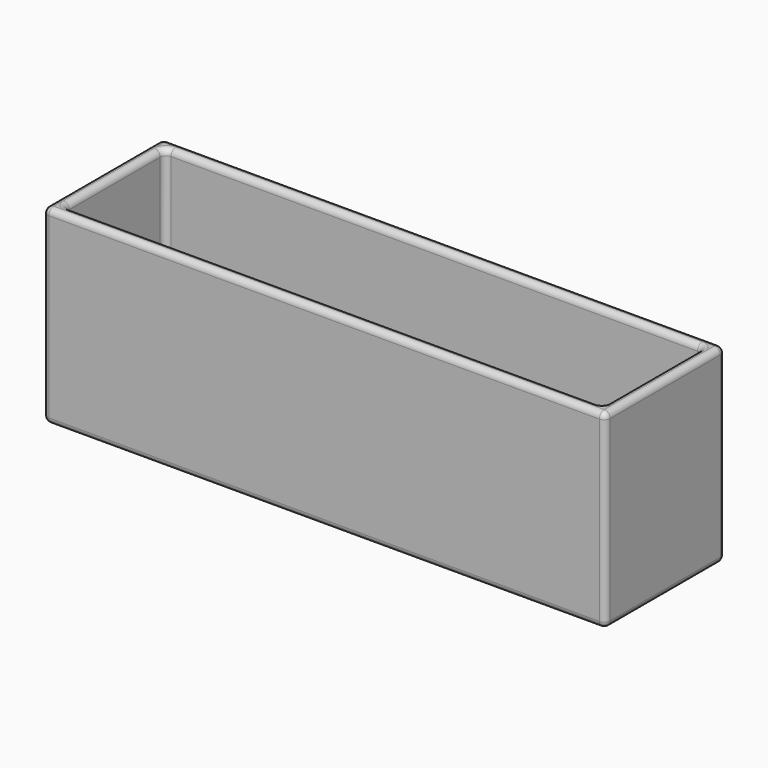
from build123d import *

# Parameters (mm, degrees)
F0_W     = 188
F0_H     = 63.5
F1_DEPTH = 50
F2_W     = 180
F2_H     = 42
F3_DEPTH = 59.5
F4_R     = 20
F5_DEPTH = 20
F6_R     = 7
F7_R     = 1.99999


# Not quite as in the source:
# - a fillet or chamfer is up to 0.001 mm smaller than in the source, because OpenCascade refuses the exact size


with BuildPart() as f1:
    # F0 (on Front) → F1 (new body)
    with BuildSketch(Plane.XZ):
        with Locations((31.2486086041, -31.75)):
            Rectangle(F0_W, F0_H)
    extrude(amount=F1_DEPTH)

    # F2 (on Top) → F3 (cut)
    with BuildSketch(Plane.XY):
        with Locations((31.2486086041, -25)):
            Rectangle(F2_W, F2_H)
    extrude(amount=-F3_DEPTH, mode=Mode.SUBTRACT)

    # F4 (on Front) → F5 (join)
    with BuildSketch(Plane.XZ):
        with Locations((31.2486086041, -31.75)):
            Circle(F4_R)
    extrude(amount=-F5_DEPTH)

    # F6
    f6_edges = [f1.edges().sort_by_distance(p)[0] for p in [
        (11.248609, 20, -31.75),
    ]]
    fillet(f6_edges, radius=F6_R)

    # F7 (radius 2 in the source; OpenCascade refuses exactly that, so slightly less here)
    f7_edges = [f1.edges().sort_by_distance(p)[0] for p in [
        (125.248609, -25, 0),
        (125.248609, -25, -63.5),
        (125.248609, 0, -31.75),
        (125.248609, -50, -31.75),
        (31.248609, 0, 0),
        (-62.751391, -50, -31.75),
        (31.248609, -50, 0),
        (-62.751391, -25, 0),
        (31.248609, -46, 0),
        (121.248609, -25, 0),
        (31.248609, -46, -59.5),
        (31.248609, 0, -63.5),
        (121.248609, -46, -29.75),
        (121.248609, -25, -59.5),
        (31.248609, -4, 0),
        (-58.751391, -25, 0),
        (121.248609, -4, -29.75),
        (31.248609, -4, -59.5),
        (31.248609, -50, -63.5),
        (-58.751391, -46, -29.75),
        (18.248609, 20, -31.75),
        (11.248609, 0, -31.75),
        (11.248609, 13, -31.75),
        (-62.751391, 0, -31.75),
        (-58.751391, -25, -59.5),
        (-58.751391, -4, -29.75),
        (-62.751391, -25, -63.5),
    ]]
    fillet(f7_edges, radius=F7_R)


solid = f1.part
